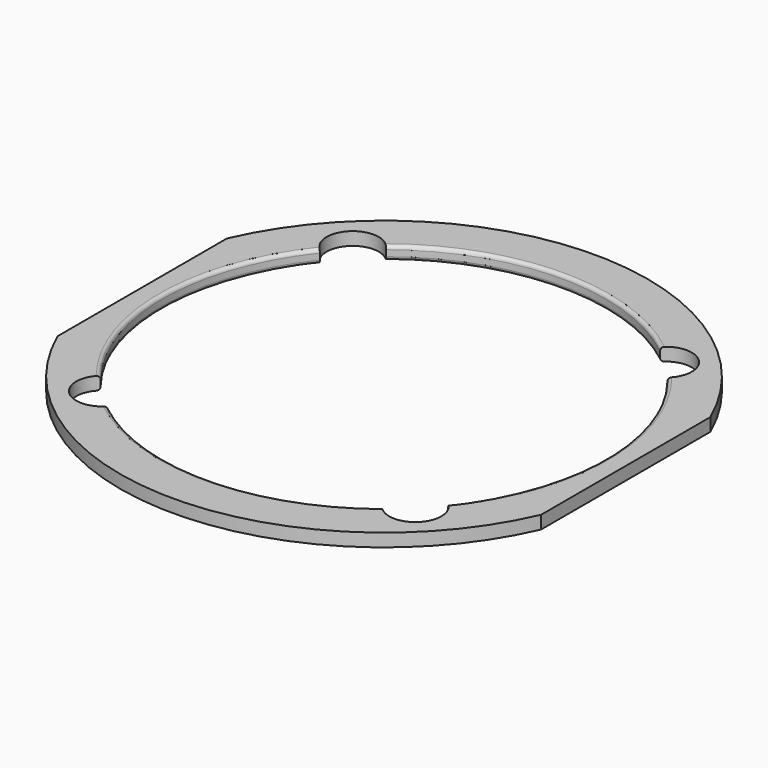
from build123d import *

# Parameters (mm, degrees)
F1_DEPTH = 19.05
F2_R     = 5.08


with BuildPart() as f1:
    # F0 (on Top) → F1 (new body)
    with BuildSketch(Plane.XY):
        with BuildLine():
            Line((-353.695, 0), (-353.695, -154.782471149))
            ThreePointArc((-353.695, -154.782471149), (0, -386.08), (353.695, -154.782471149))
            Line((353.695, -154.782471149), (353.695, 0))
            Line((353.695, 0), (353.695, 154.782471149))
            ThreePointArc((353.695, 154.782471149), (0, 386.08), (-353.695, 154.782471149))
            Line((-353.695, 154.782471149), (-353.695, 0))
        make_face()
        with BuildLine():
            ThreePointArc((254.3058976541, 200.51766236), (305.9704131573, 106.1175233991), (323.85, 0))
            ThreePointArc((323.85, 0), (305.9704131573, -106.1175233991), (254.3058976541, -200.51766236))
            ThreePointArc((254.3058976541, -200.51766236), (255.9372994505, -255.9372994505), (200.51766236, -254.3058976541))
            ThreePointArc((200.51766236, -254.3058976541), (0, -323.85), (-200.51766236, -254.3058976541))
            ThreePointArc((-200.51766236, -254.3058976541), (-255.9372994505, -255.9372994505), (-254.3058976541, -200.51766236))
            ThreePointArc((-254.3058976541, -200.51766236), (-323.85, 0), (-254.3058976541, 200.51766236))
            ThreePointArc((-254.3058976541, 200.51766236), (-255.9372994505, 255.9372994505), (-200.51766236, 254.3058976541))
            ThreePointArc((-200.51766236, 254.3058976541), (0, 323.85), (200.51766236, 254.3058976541))
            ThreePointArc((200.51766236, 254.3058976541), (255.9372994505, 255.9372994505), (254.3058976541, 200.51766236))
        make_face(mode=Mode.SUBTRACT)
    extrude(amount=F1_DEPTH)

    # F2
    f2_edges = [f1.edges().sort_by_distance(p)[0] for p in [
        (0, 323.85, 19.05),
        (323.85, 0, 19.05),
        (0, 323.85, 0),
        (323.85, 0, 0),
        (0, -323.85, 19.05),
        (-323.85, 0, 19.05),
        (-323.85, 0, 0),
        (0, -323.85, 0),
    ]]
    fillet(f2_edges, radius=F2_R)


solid = f1.part
